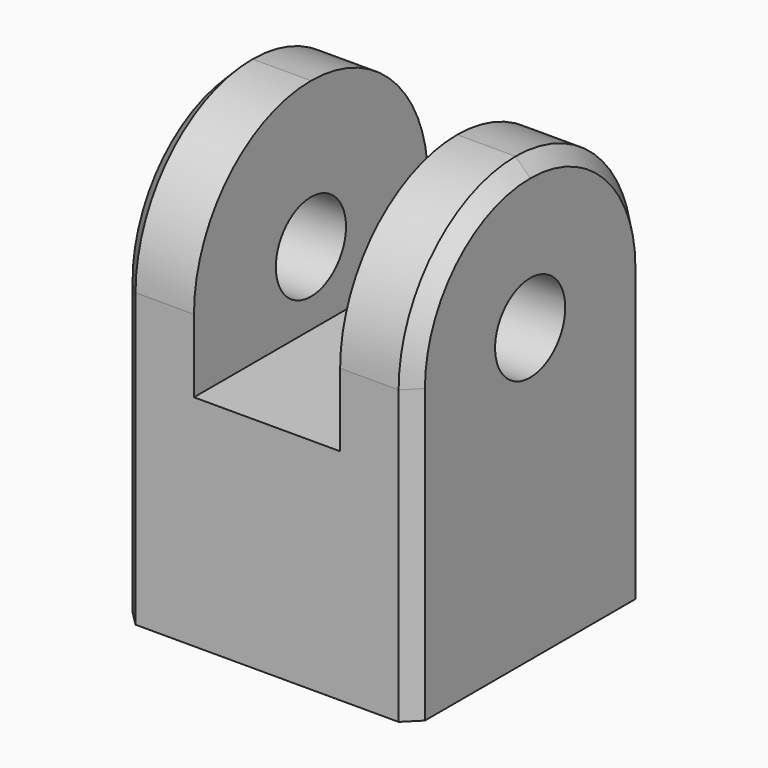
from build123d import *

# Parameters (mm, degrees)
F0_W          = 40
F0_H          = 40
F1_DEPTH      = 60
F2_W          = 20
F2_H          = 40
F3_DEPTH      = 30
F4_R          = 19.99999
F5_SIZE       = 2
F6_R          = 6
F7_DEPTH      = 56.6
F7_DEPTH_BACK = 25


# Not quite as in the source:
# - a fillet or chamfer is up to 0.001 mm smaller than in the source, because OpenCascade refuses the exact size


with BuildPart() as f1:
    # F0 (on Top) → F1 (new body)
    with BuildSketch(Plane.XY):
        Rectangle(F0_W, F0_H)
    extrude(amount=F1_DEPTH)

    # F2 (on face) → F3 (cut)
    with BuildSketch(Plane.XY.offset(60)):
        Rectangle(F2_W, F2_H)
    extrude(amount=-F3_DEPTH, mode=Mode.SUBTRACT)

    # F4 (radius 20 in the source; OpenCascade refuses exactly that, so slightly less here)
    f4_edges = [f1.edges().sort_by_distance(p)[0] for p in [
        (15, -20, 60),
        (-15, -20, 60),
        (15, 20, 60),
        (-15, 20, 60),
    ]]
    fillet(f4_edges, radius=F4_R)

    # F5
    f5_edges = [f1.edges().sort_by_distance(p)[0] for p in [
        (-20, -20, 20.000005),
        (-20, -14.142139, 54.142139),
        (20, -14.142139, 54.142139),
    ]]
    chamfer(f5_edges, length=F5_SIZE)

    # F6 (on face) → F7 (cut, two sides)
    with BuildSketch(Plane.YZ.offset(20)) as f7_sk:
        with Locations((0, 40)):
            Circle(F6_R)
    extrude(amount=-F7_DEPTH, mode=Mode.SUBTRACT)
    extrude(f7_sk.sketch, amount=F7_DEPTH_BACK, mode=Mode.SUBTRACT)


solid = f1.part
